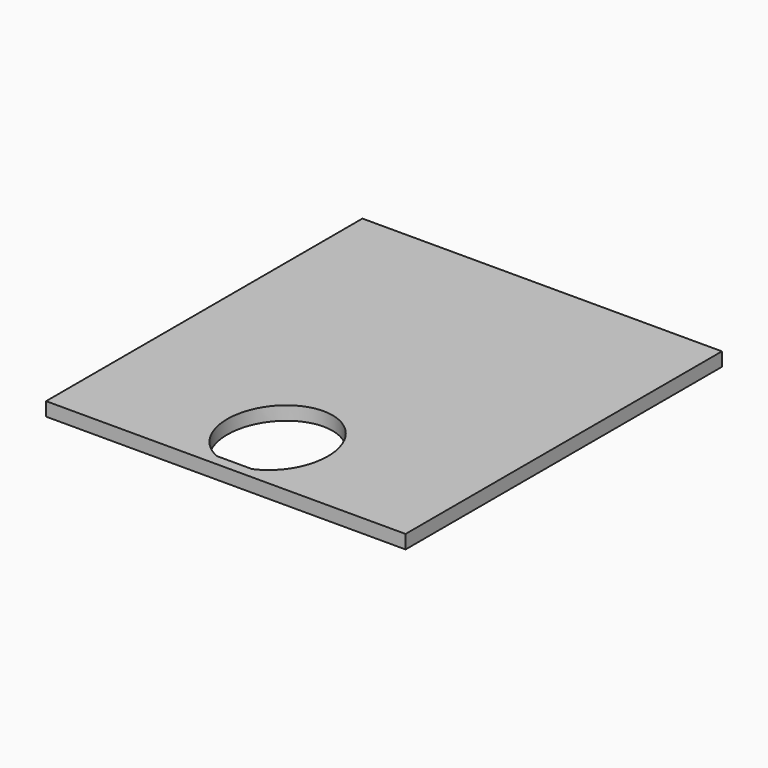
from build123d import *

# Parameters (mm, degrees)
F0_W     = 304.8
F0_H     = 335.28
F1_DEPTH = 11.5824
F3_DEPTH = 11.5834


with BuildPart() as f1:
    # F0 (on Top) → F1 (new body)
    with BuildSketch(Plane.XY):
        Rectangle(F0_W, F0_H)
    extrude(amount=F1_DEPTH)

    # F2 (on face) → F3 (cut, through all)
    with BuildSketch(Plane.XY.offset(11.5824)):
        with BuildLine():
            Line((-14.8492275557, -158.496), (14.8492275557, -158.496))
            add(Edge.make_bspline(
                [(14.8492275557, -158.496), (68.3482837309, -135.801132311), (34.1741418655, -83.5709657846), (0, -31.3407992582), (-34.1741418655, -83.5709657846), (-68.3482837309, -135.801132311), (-14.8492275557, -158.496)],
                knots=[3.4970138553, 3.4970138553, 3.4970138553, 5.3544614899, 5.3544614899, 7.2119091245, 7.2119091245, 9.0693567591, 9.0693567591, 9.0693567591], degree=2, weights=[1, 0.5988565087, 1, 0.5988565087, 1, 0.5988565087, 1]))
        make_face()
    extrude(amount=-F3_DEPTH, mode=Mode.SUBTRACT)


solid = f1.part
